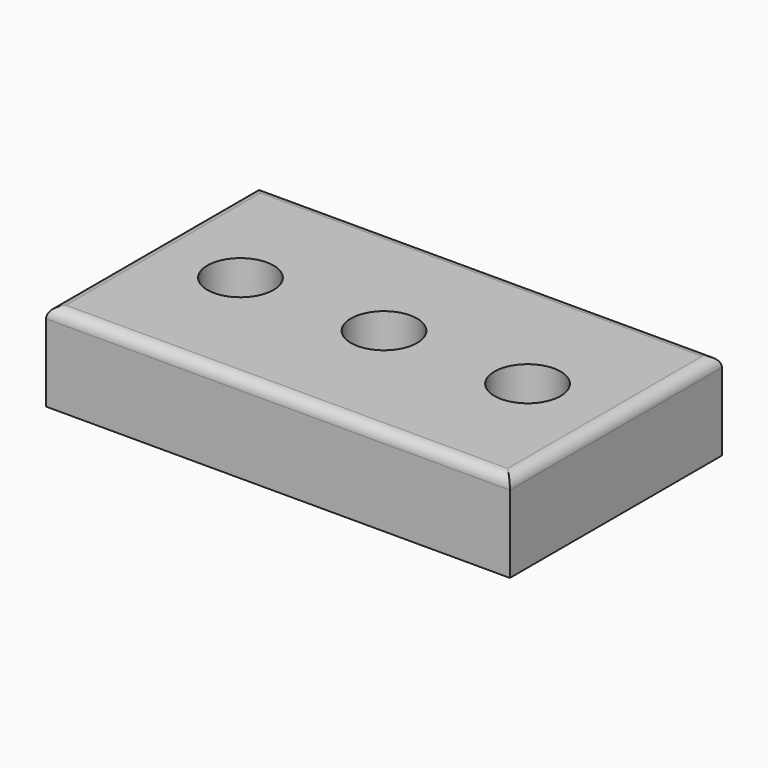
from build123d import *

# Parameters (mm, degrees)
F0_W     = 105
F0_H     = 60
F0_R     = 7.5
F1_DEPTH = 20
F2_DEPTH = 5
F3_R     = 2.5


with BuildPart() as f1:
    # F0 (on Top) → F1 (new body)
    with BuildSketch(Plane.XY):
        Rectangle(F0_W, F0_H)
        with Locations((-32.5, 0)):
            Circle(F0_R, mode=Mode.SUBTRACT)
        with BuildLine():
            ThreePointArc((-7.5, 0), (0, 7.5), (7.5, 0))
            ThreePointArc((7.5, 0), (0, -7.5), (-7.5, 0))
        make_face(mode=Mode.SUBTRACT)
        with BuildLine():
            ThreePointArc((40, 0), (32.5, -7.5), (25, 0))
            ThreePointArc((25, 0), (32.5, 7.5), (40, 0))
        make_face(mode=Mode.SUBTRACT)
    extrude(amount=F1_DEPTH)

    # F3
    f3_edges = [f1.edges().sort_by_distance(p)[0] for p in [
        (0, -30, 20),
        (-52.5, 0, 20),
        (0, 30, 20),
        (52.5, 0, 20),
    ]]
    fillet(f3_edges, radius=F3_R)


with BuildPart() as f2:
    # F0 (on Top) → F2 (new body)
    with BuildSketch(Plane.XY):
        with BuildLine():
            ThreePointArc((-7.5, 0), (0, -7.5), (7.5, 0))
            ThreePointArc((7.5, 0), (0, 7.5), (-7.5, 0))
        make_face()
    extrude(amount=F2_DEPTH)


with BuildPart() as f2b:
    # F0 (on Top) → F2, piece 2 (new body)
    with BuildSketch(Plane.XY):
        with Locations((-32.5, 0)):
            Circle(F0_R)
    extrude(amount=F2_DEPTH)


with BuildPart() as f2c:
    # F0 (on Top) → F2, piece 3 (new body)
    with BuildSketch(Plane.XY):
        with BuildLine():
            ThreePointArc((40, 0), (32.5, 7.5), (25, 0))
            ThreePointArc((25, 0), (32.5, -7.5), (40, 0))
        make_face()
    extrude(amount=F2_DEPTH)


solid = Compound([f1.part, f2.part, f2b.part, f2c.part])
